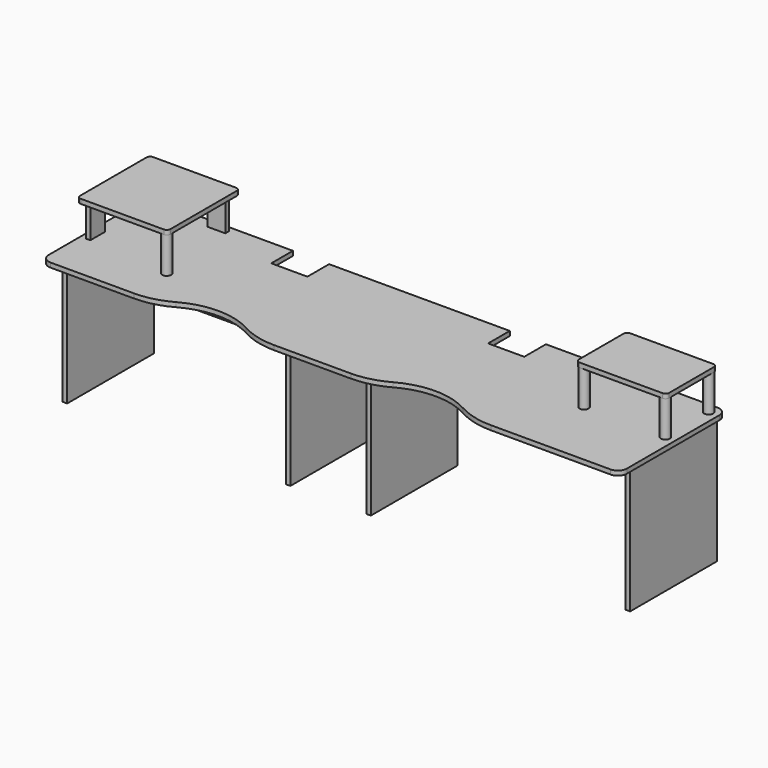
from build123d import *

# Parameters (mm, degrees)
F2_DEPTH  = 25
F3_R      = 400
F6_W      = 25
F6_H      = 630
F7_DEPTH  = 705
F8_W      = 25
F8_H      = 200
F9_DEPTH  = 60
F10_W     = 500
F10_H     = 200
F11_DEPTH = 25
F12_W     = 3200
F12_H     = 30
F13_DEPTH = 705.001
F14_R     = 50
F15_W     = 100
F15_H     = 25
F16_DEPTH = 200
F15_W_2   = 25
F15_H_2   = 100
F15_R     = 25
F17_W     = 500
F17_H     = 500
F18_DEPTH = 25
F19_R     = 20
F21_DEPTH = 25
F20_W     = 420
F20_H     = 400
F22_R     = 25
F23_DEPTH = 200
F24_W     = 500
F24_H     = 350
F25_DEPTH = 25
F26_R     = 20


# Not quite as in the source:
# - a pattern or mirror of a feature is missing from the dataset's text; its kind, count and spacing are read off the source's solid


with BuildPart() as f2:
    # F1 (on Top) → F2 (new body)
    with BuildSketch(Plane.XY):
        with BuildLine():
            Line((800, 0), (0, 0))
            Line((0, 0), (0, -740))
            Line((0, -740), (635.4248688935, -740))
            ThreePointArc((635.4248688935, -740), (900, -640), (1164.5751311065, -740))
            Line((1164.5751311065, -740), (1835.4248688935, -740))
            ThreePointArc((1835.4248688935, -740), (2100, -640), (2364.5751311065, -740))
            Line((2364.5751311065, -740), (3200, -740))
            Line((3200, -740), (3200, 0))
            Line((3200, 0), (2200, 0))
            Line((2200, 0), (2200, -150))
            Line((2200, -150), (2000, -150))
            Line((2000, -150), (2000, 0))
            Line((2000, 0), (1000, 0))
            Line((1000, 0), (1000, -150))
            Line((1000, -150), (800, -150))
            Line((800, -150), (800, 0))
        make_face()
    extrude(amount=-F2_DEPTH)

    # F3
    f3_edges = [f2.edges().sort_by_distance(p)[0] for p in [
        (635.424869, -740, -12.5),
        (1164.575131, -740, -12.5),
        (1835.424869, -740, -12.5),
        (2364.575131, -740, -12.5),
    ]]
    fillet(f3_edges, radius=F3_R)

    # F6 (on face) → F7 (join)
    with BuildSketch(Plane(origin=(0, 0, -25), x_dir=(1, 0, 0), z_dir=(0, 0, -1))):
        with Locations((1277.5, 315)):
            Rectangle(F6_W, F6_H)
        with Locations((1722.5, 315)):
            Rectangle(F6_W, F6_H)
        with Locations((42.5, 315)):
            Rectangle(F6_W, F6_H)
        with Locations((3157.5, 315)):
            Rectangle(F6_W, F6_H)
    extrude(amount=F7_DEPTH)

    # F8 (on face) → F9 (join)
    with BuildSketch(Plane(origin=(0, 0, -25), x_dir=(1, 0, 0), z_dir=(0, 0, -1))):
        with Locations((662.5, 100)):
            Rectangle(F8_W, F8_H)
        with Locations((1137.5, 100)):
            Rectangle(F8_W, F8_H)
    f9 = extrude(amount=F9_DEPTH)

    # F9_copies: F9 across plane
    add(f9.mirror(Plane(origin=(1500, 0, 0), x_dir=(0, 0, 1), z_dir=(1, 0, 0))))

    # F10 (on face) → F11 (join)
    with BuildSketch(Plane(origin=(0, 0, -85), x_dir=(1, 0, 0), z_dir=(0, 0, -1))):
        with Locations((900, 100)):
            Rectangle(F10_W, F10_H)
    f11 = extrude(amount=F11_DEPTH)

    # F11_copies: F11 across plane
    add(f11.mirror(Plane(origin=(1500, 0, 0), x_dir=(0, 0, 1), z_dir=(1, 0, 0))))

    # F12 (on face) → F13 (cut, through all)
    with BuildSketch(Plane(origin=(0, 0, -25), x_dir=(1, 0, 0), z_dir=(0, 0, -1))):
        with Locations((1600, 15)):
            Rectangle(F12_W, F12_H)
    extrude(amount=F13_DEPTH, mode=Mode.SUBTRACT)

    # F14
    f14_edges = [f2.edges().sort_by_distance(p)[0] for p in [
        (3200, -740, -12.5),
        (3200, 0, -12.5),
        (0, 0, -12.5),
        (0, -740, -12.5),
    ]]
    fillet(f14_edges, radius=F14_R)


with BuildPart() as f16:
    # F15 (on face) → F16 (new body)
    with BuildSketch(Plane.XY):
        with Locations((140, -42.5)):
            Rectangle(F15_W, F15_H)
    extrude(amount=F16_DEPTH)


with BuildPart() as f16b:
    # F15 (on face) → F16, piece 2 (new body)
    with BuildSketch(Plane.XY):
        with Locations((42.5, -140)):
            Rectangle(F15_W_2, F15_H_2)
    extrude(amount=F16_DEPTH)


with BuildPart() as f16c:
    # F15 (on face) → F16, piece 3 (new body)
    with BuildSketch(Plane.XY):
        with Locations((420, -42.5)):
            Rectangle(F15_W, F15_H)
    extrude(amount=F16_DEPTH)


with BuildPart() as f16d:
    # F15 (on face) → F16, piece 4 (new body)
    with BuildSketch(Plane.XY):
        with Locations((42.5, -420)):
            Rectangle(F15_W_2, F15_H_2)
    extrude(amount=F16_DEPTH)


with BuildPart() as f16e:
    # F15 (on face) → F16, piece 5 (new body)
    with BuildSketch(Plane.XY):
        with Locations((505, -505)):
            Circle(F15_R)
    extrude(amount=F16_DEPTH)


with BuildPart() as f18:
    # F17 (on face) → F18 (new body)
    with BuildSketch(Plane.XY.offset(200)):
        with Locations((280, -280)):
            Rectangle(F17_W, F17_H)
    extrude(amount=F18_DEPTH)

    # F19
    f19_edges = [f18.edges().sort_by_distance(p)[0] for p in [
        (530, -530, 212.5),
        (530, -30, 212.5),
        (30, -530, 212.5),
        (30, -30, 212.5),
    ]]
    fillet(f19_edges, radius=F19_R)


with BuildPart() as f21:
    # F20 (on face) → F21 (new body)
    with BuildSketch(Plane(origin=(0, -30, 0), x_dir=(-1, 0, 0), z_dir=(0, 1, 0))):
        Polygon((-1265, -425), (-55, -425), (-55, -25), (-650, -25), (-650, -110), (-1150, -110), (-1150, -25), (-1265, -25), align=None)
    extrude(amount=-F21_DEPTH)


with BuildPart() as f21b:
    # F20 (on face) → F21, piece 2 (new body)
    with BuildSketch(Plane(origin=(0, -30, 0), x_dir=(-1, 0, 0), z_dir=(0, 1, 0))):
        with Locations((-1500, -225)):
            Rectangle(F20_W, F20_H)
    extrude(amount=-F21_DEPTH)


with BuildPart() as f21c:
    # F20 (on face) → F21, piece 3 (new body)
    with BuildSketch(Plane(origin=(0, -30, 0), x_dir=(-1, 0, 0), z_dir=(0, 1, 0))):
        Polygon((-2350, -25), (-3145, -25), (-3145, -425), (-1735, -425), (-1735, -25), (-1850, -25), (-1850, -110), (-2350, -110), align=None)
    extrude(amount=-F21_DEPTH)


with BuildPart() as f23:
    # F22 (on face) → F23 (new body)
    with BuildSketch(Plane.XY):
        with Locations((2695, -55)):
            Circle(F22_R)
    extrude(amount=F23_DEPTH)


with BuildPart() as f23b:
    # F22 (on face) → F23, piece 2 (new body)
    with BuildSketch(Plane.XY):
        with Locations((3145, -55)):
            Circle(F22_R)
    extrude(amount=F23_DEPTH)


with BuildPart() as f23c:
    # F22 (on face) → F23, piece 3 (new body)
    with BuildSketch(Plane.XY):
        with Locations((3145, -355)):
            Circle(F22_R)
    extrude(amount=F23_DEPTH)


with BuildPart() as f23d:
    # F22 (on face) → F23, piece 4 (new body)
    with BuildSketch(Plane.XY):
        with Locations((2695, -355)):
            Circle(F22_R)
    extrude(amount=F23_DEPTH)


with BuildPart() as f25:
    # F24 (on face) → F25 (new body)
    with BuildSketch(Plane.XY.offset(200)):
        with Locations((2920, -205)):
            Rectangle(F24_W, F24_H)
    extrude(amount=F25_DEPTH)

    # F26
    f26_edges = [f25.edges().sort_by_distance(p)[0] for p in [
        (2670, -380, 212.5),
        (3170, -380, 212.5),
        (2670, -30, 212.5),
        (3170, -30, 212.5),
    ]]
    fillet(f26_edges, radius=F26_R)


solid = Compound([f2.part, f16.part, f16b.part, f16c.part, f16d.part, f16e.part, f18.part, f21.part, f21b.part, f21c.part, f23.part, f23b.part, f23c.part, f23d.part, f25.part])
